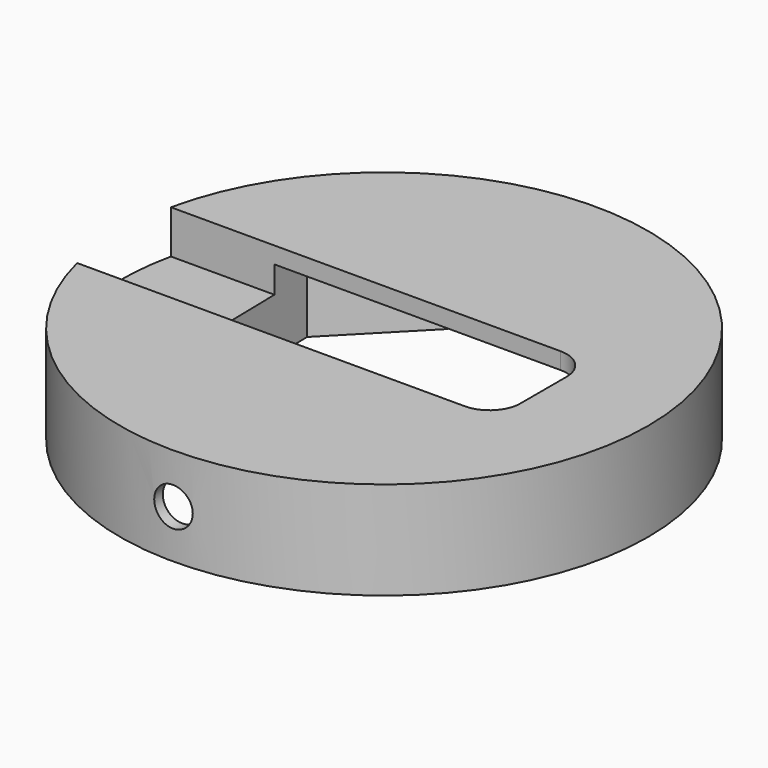
from build123d import *

# Parameters (mm, degrees)
F0_R          = 68.5
F1_DEPTH      = 25.4
F3_DEPTH      = 11.25
F6_DEPTH      = 21.082
F4_R          = 5
F7_DEPTH      = 68.501
F7_DEPTH_BACK = 68.501


with BuildPart() as f1:
    # F0 (on Top) → F1 (new body)
    with BuildSketch(Plane.XY):
        Circle(F0_R)
    extrude(amount=F1_DEPTH)

    # F2 (on face) → F3 (cut)
    with BuildSketch(Plane.XY.offset(25.4)):
        with BuildLine():
            Line((34.15, 14.5270901566), (-88.2992463768, 14.5270901566))
            Line((-88.2992463768, 14.5270901566), (-88.2992463768, -16.4609098434))
            Line((-88.2992463768, -16.4609098434), (34.15, -16.4609098434))
            ThreePointArc((34.15, -16.4609098434), (39.8068542495, -14.1177640929), (42.15, -8.4609098434))
            Line((42.15, -8.4609098434), (42.15, 6.5270901566))
            ThreePointArc((42.15, 6.5270901566), (39.8068542495, 12.183944406), (34.15, 14.5270901566))
        make_face()
    extrude(amount=-F3_DEPTH, mode=Mode.SUBTRACT)

    # F5 (on face) → F6 (cut)
    with BuildSketch(Plane(origin=(0, 0, 0), x_dir=(1, 0, 0), z_dir=(0, 0, -1))):
        Polygon((10.1280519739, 65.532), (-9.8341628909, 65.532), (-25.9055476636, 45.72), (-39.7767797112, 25.4), (-39.7767797112, 0), (-40.3115227818, -25.4), (-20.4457305372, -45.72), (-10.3001166135, -65.532), (9.6642833865, -65.532), (32.5386694628, -45.72), (48.4360772182, -25.4), (48.9794053137, 0), (48.9794053137, 25.4), (27.0890761167, 45.72), align=None)
    extrude(amount=-F6_DEPTH, mode=Mode.SUBTRACT)

    # F4 (on Front) → F7 (cut, two sides)
    with BuildSketch(Plane.XZ) as f7_sk:
        with Locations((0, 12.5027870712)):
            Circle(F4_R)
    extrude(amount=-F7_DEPTH, mode=Mode.SUBTRACT)
    extrude(f7_sk.sketch, amount=F7_DEPTH_BACK, mode=Mode.SUBTRACT)


solid = f1.part
